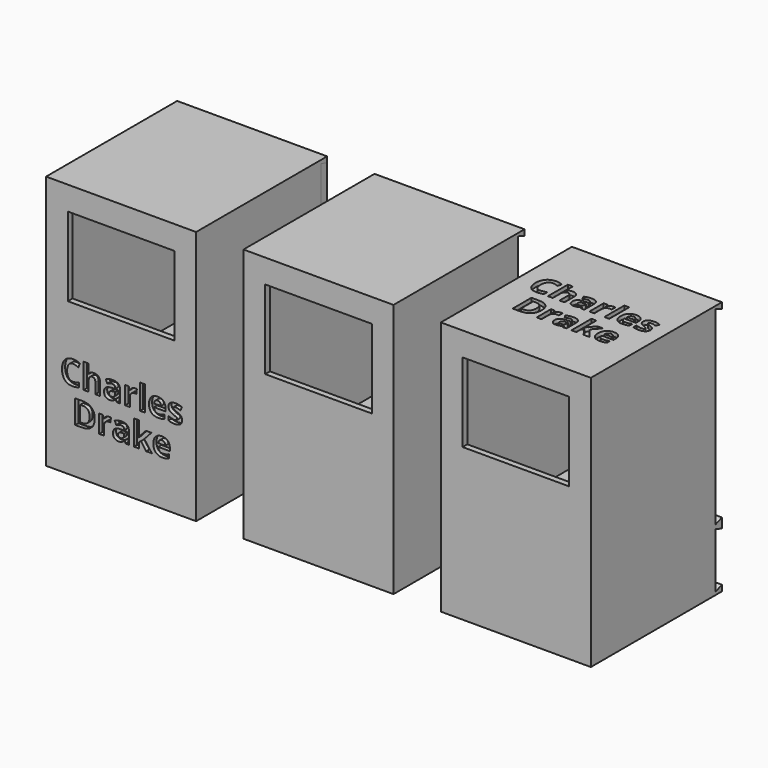
from build123d import *

# Parameters (mm, degrees)
F0_W          = 76
F0_H          = 83
F0_W_2        = 70
F0_H_2        = 77
F1_DEPTH      = 99
F2_T          = -3
F3_DEPTH      = 30
F4_T          = -3
F5_W          = 54
F5_H          = 40
F6_DEPTH      = 3
F8_DEPTH      = 73
F9_DEPTH      = 2
F11_DEPTH     = 73
F13_DEPTH     = 73
F15_DEPTH     = 73
F17_DEPTH     = 2.5
F18_T2_ANGLE  = 180
F20_DEPTH     = 2.5
F21_T2_ANGLE  = 180
F23_TEXT_SIZE = 16.6666666667
F24_DEPTH     = 2
F26_TEXT_SIZE = 16.6666666667
F27_DEPTH     = 2


# Not quite as in the source:
# - a fillet or chamfer that OpenCascade refuses, or shapes differently, is made with other operations: its cross-section is extruded or revolved along the edge and cut away or added
# - a feature names something its author has since deleted; it is built from what else it names
# - Text() gives the source's letters only with a copy of the font that has no kerning and outlines rounded to 1/6400 em; it was checked with that copy


with BuildPart() as f1:
    # F0 (on Top) → F1 (new body)
    with BuildSketch(Plane.XY):
        Rectangle(F0_W, F0_H)
        Rectangle(F0_W_2, F0_H_2, mode=Mode.SUBTRACT)
        Rectangle(F0_W_2, F0_H_2)
    extrude(amount=F1_DEPTH)

    # F2
    f2_openings = [f1.faces().sort_by_distance(p)[0] for p in [
        (0, 41.5, 49.5),
    ]]
    offset(amount=F2_T, openings=f2_openings)

    # F3 (add): a face of the model
    f3_faces = [f1.faces().sort_by_distance(p)[0] for p in [
        (0, 0, 0),
    ]]
    extrude(f3_faces, amount=F3_DEPTH)

    # F4: a shell. OpenCascade refuses it in one call, so the cavity is built on its own and cut out:
    # the body offset inwards by the wall thickness, plus a prism from it out through each open face.
    f4_core = offset(f1.part, amount=F4_T, kind=Kind.INTERSECTION, mode=Mode.PRIVATE)
    f4_exits = [f4_core.faces().sort_by_distance(p)[0] for p in [
        (0, 38.5, -13.5),
    ]]
    add(f4_core, mode=Mode.SUBTRACT)
    extrude(f4_exits, amount=-F4_T, mode=Mode.SUBTRACT)

    # F5 (on face) → F6 (cut, through all)
    with BuildSketch(Plane.XZ.offset(41.5)):
        with Locations((0, 67)):
            Rectangle(F5_W, F5_H)
    extrude(amount=-F6_DEPTH, mode=Mode.SUBTRACT)

    # F7 (on face) → F8 (cut, through all)
    with BuildSketch(Plane.YZ.offset(38)):
        Polygon((41.5, 3), (41.5, 96), (37.5, 97.5), (37.5, 1.5), align=None)
    extrude(amount=-F8_DEPTH, mode=Mode.SUBTRACT)

    # F9 (add): a face of the model
    f9_faces = [f1.faces().sort_by_distance(p)[0] for p in [
        (0, 1.5, 0),
    ]]
    extrude(f9_faces, amount=F9_DEPTH)

    # F10 (on face) → F11 (cut, through all)
    with BuildSketch(Plane.YZ.offset(38)):
        Polygon((41.5, -27), (41.5, -2), (37.5, -0.5), (37.5, -28.5), align=None)
    extrude(amount=-F11_DEPTH, mode=Mode.SUBTRACT)


with BuildPart() as f13:
    # F12 (on face) → F13 (new body, through all)
    with BuildSketch(Plane.YZ.offset(38)):
        Polygon((41.5, 3.5), (41.5, 96), (37.5, 97.5), (37.5, 2), align=None)
    extrude(amount=-F13_DEPTH)

    # F16 (on face) → F17 (cut)
    with BuildSketch(Plane(origin=(0, 41.5, 0), x_dir=(-1, 0, 0), z_dir=(0, 1, 0))):
        with BuildLine():
            Line((-33, 59.5), (-33, 39.5))
            ThreePointArc((-33, 39.5), (-23, 49.5), (-33, 59.5))
        make_face()
    extrude(amount=-F17_DEPTH, mode=Mode.SUBTRACT)

    # F18: fillet of radius 5 on 1 edges, made by hand

    # F18_s1 → F18_t2 (revolve)
    with BuildSketch(Plane.YZ.offset(33)):
        with BuildLine():
            ThreePointArc((41.5, 39.5), (39.6698729811, 41.3301270189), (39, 43.8301270189))
            Line((39, 43.8301270189), (39, 39.5))
            Line((39, 39.5), (41.5, 39.5))
        make_face()
    revolve(axis=Axis((33, 39, 49.5), (0, 1, 0)), revolution_arc=F18_T2_ANGLE)


with BuildPart() as f15:
    # F14 (on face) → F15 (new body, through all)
    with BuildSketch(Plane.YZ.offset(38)):
        Polygon((41.5, -26.5), (41.5, -2), (37.5, -0.5), (37.5, -28), align=None)
    extrude(amount=-F15_DEPTH)

    # F19 (on face) → F20 (cut)
    with BuildSketch(Plane(origin=(0, 41.5, 0), x_dir=(-1, 0, 0), z_dir=(0, 1, 0))):
        with BuildLine():
            Line((-33, -4.5000000002), (-33, -24.5000000002))
            ThreePointArc((-33, -24.5000000002), (-23, -14.5000000002), (-33, -4.5000000002))
        make_face()
    extrude(amount=-F20_DEPTH, mode=Mode.SUBTRACT)

    # F21: fillet of radius 5 on 1 edges, made by hand

    # F21_s1 → F21_t2 (revolve)
    with BuildSketch(Plane.YZ.offset(33)):
        with BuildLine():
            ThreePointArc((41.5, -24.5000000002), (39.6698729811, -22.6698729812), (39, -20.1698729812))
            Line((39, -20.1698729812), (39, -24.5000000002))
            Line((39, -24.5000000002), (41.5, -24.5000000002))
        make_face()
    revolve(axis=Axis((33, 39, -14.5000000002), (0, 1, 0)), revolution_arc=F21_T2_ANGLE)


with BuildPart() as f22_1:
    # F22: copy of F1
    add(f1.part.moved(Location((100, 0, 0))))


with BuildPart() as f1_1:
    add(f1.part)

    # F23 (on face) → F24 (cut)
    with BuildSketch(Plane.XZ.offset(41.5)):
        with Locations((-30.8958333333, 10)):
            Text('Charles', F23_TEXT_SIZE, font='Open Sans', font_style=FontStyle.BOLD, text_align=(TextAlign.LEFT, TextAlign.BOTTOM))
        with Locations((-24.7200520833, -7)):
            Text('Drake', F23_TEXT_SIZE, font='Open Sans', font_style=FontStyle.BOLD, text_align=(TextAlign.LEFT, TextAlign.BOTTOM))
    extrude(amount=-F24_DEPTH, mode=Mode.SUBTRACT)


with BuildPart() as f25_1:
    # F25: copy of F22_1
    add(f22_1.part.moved(Location((100, 0, 0))))

    # F26 (on face) → F27 (cut)
    with BuildSketch(Plane.XY.offset(99)):
        with Locations((169.1041666667, 2.5)):
            Text('Charles', F26_TEXT_SIZE, font='Open Sans', font_style=FontStyle.BOLD, text_align=(TextAlign.LEFT, TextAlign.BOTTOM))
        with Locations((175.2799479167, -14.5)):
            Text('Drake', F26_TEXT_SIZE, font='Open Sans', font_style=FontStyle.BOLD, text_align=(TextAlign.LEFT, TextAlign.BOTTOM))
    extrude(amount=-F27_DEPTH, mode=Mode.SUBTRACT)


solid = Compound([f13.part, f15.part, f22_1.part, f1_1.part, f25_1.part])
